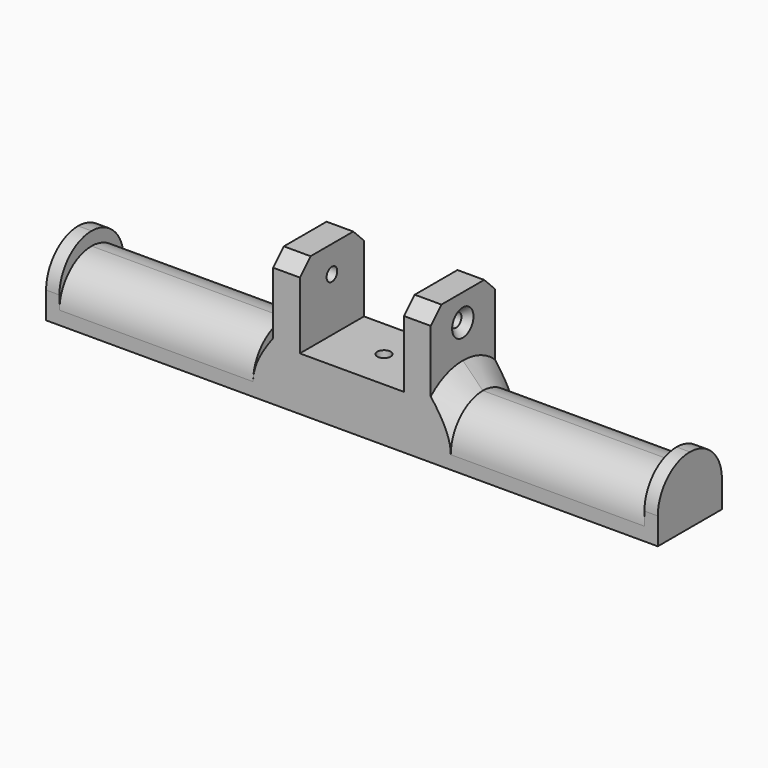
from build123d import *

# Parameters (mm, degrees)
F1_DEPTH     = 30
F2_R         = 14.99999
F4_DEPTH     = 219.001
F5_T1_DEPTH  = 2e-05
F5_T6_ANGLE  = 163.702935025
F5_T12_ANGLE = 163.702935025
F5_T18_ANGLE = 163.702935025
F5_T24_ANGLE = 163.702935025
F6_SIZE      = 5
F7_R         = 2.5
F8_DEPTH     = 139.001
F9_W         = 20
F9_H         = 20
F11_R        = 2.5
F12_DEPTH    = 20.001
F13_SIZE     = 2.5
F14_W        = 5
F14_H        = 25
F15_DEPTH    = 30
F16_R        = 14.99999
F17_R        = 5
F18_DEPTH    = 7.5
F19_SIZE     = 2.49999


# Not quite as in the source:
# - a fillet or chamfer that OpenCascade refuses, or shapes differently, is made with other operations: its cross-section is extruded or revolved along the edge and cut away or added
# - a fillet or chamfer is up to 0.001 mm smaller than in the source, because OpenCascade refuses the exact size


with BuildPart() as f1:
    # F0 (on Front) → F1 (new body)
    with BuildSketch(Plane.XZ):
        Polygon((-109.5, 0), (0, 0), (109.5, 0), (109.5, 20), (29.5, 20), (29.5, 50), (19.5, 50), (19.5, 20), (0, 20), (-19.5, 20), (-19.5, 50), (-29.5, 50), (-29.5, 20), (-109.5, 20), align=None)
    extrude(amount=F1_DEPTH)

    # F2 (radius 15 in the source; OpenCascade refuses exactly that, so slightly less here)
    f2_edges = [f1.edges().sort_by_distance(p)[0] for p in [
        (-69.5, 0, 20),
        (-69.5, -30, 20),
        (69.5, 0, 20),
        (69.5, -30, 20),
    ]]
    fillet(f2_edges, radius=F2_R)

    # F3 (on face) → F4 (cut, through all)
    with BuildSketch(Plane(origin=(-109.5, 0, 0), x_dir=(0, -1, 0), z_dir=(-1, 0, 0))):
        with BuildLine():
            Line((25, 0), (25, 5))
            ThreePointArc((25, 5), (15, 15), (5, 5))
            Line((5, 5), (5, 0))
            Line((5, 0), (25, 0))
        make_face()
    extrude(amount=-F4_DEPTH, mode=Mode.SUBTRACT)

    # F5: chamfer of 7.5 on 4 edges, made by hand

    # F5_s2 → F5_t1 (join)
    with BuildSketch(Plane.XZ.offset(14.99999)):
        Polygon((-37, 20), (-29.5, 27.5), (-29.5, 20), align=None)
        Polygon((37, 20), (29.5, 27.5), (29.5, 20), align=None)
    extrude(amount=F5_T1_DEPTH)


with BuildPart() as f5_tool4:
    # F5_s5 → F5_t6 (revolve)
    with BuildSketch(Plane(origin=(0, -12.4720838446, -3.6463990318), x_dir=(1, 0, 0), z_dir=(0, -0.9598196681, -0.2806175417))):
        Polygon((-37, -5.9916217418), (-29.5, -13.4916217418), (-29.5, -5.9916217418), align=None)
    revolve(axis=Axis((-29.5, -14.99999, 5.00001), (1, 0, 0)), revolution_arc=F5_T6_ANGLE)

    split(bisect_by=Plane.XZ, keep=Keep.TOP)

    split(bisect_by=Plane.XY, keep=Keep.TOP)


with BuildPart() as f1_1:
    add(f1.part)

    # F5_t3: union F5_tool4
    add(f5_tool4.part)


with BuildPart() as f5_tool10:
    # F5_s11 → F5_t12 (revolve)
    with BuildSketch(Plane(origin=(0, -12.4720838446, -3.6463990318), x_dir=(1, 0, 0), z_dir=(0, -0.9598196681, -0.2806175417))):
        Polygon((29.5, -13.4916217418), (37, -5.9916217418), (29.5, -5.9916217418), align=None)
    revolve(axis=Axis((29.5, -14.99999, 5.00001), (1, 0, 0)), revolution_arc=F5_T12_ANGLE)

    split(bisect_by=Plane.XZ, keep=Keep.TOP)

    split(bisect_by=Plane.XY, keep=Keep.TOP)


with BuildPart() as f1_2:
    add(f1_1.part)

    # F5_t9: union F5_tool10
    add(f5_tool10.part)


with BuildPart() as f5_tool16:
    # F5_s17 → F5_t18 (revolve)
    with BuildSketch(Plane.XZ.offset(15.00001)):
        Polygon((37, 20), (29.5, 27.5), (29.5, 20), align=None)
    revolve(axis=Axis((29.5, -15.00001, 5.00001), (1, 0, 0)), revolution_arc=F5_T18_ANGLE)

    split(bisect_by=Plane.XY, keep=Keep.TOP)

    split(bisect_by=Plane.XZ.offset(30), keep=Keep.BOTTOM)


with BuildPart() as f1_3:
    add(f1_2.part)

    # F5_t15: union F5_tool16
    add(f5_tool16.part)


with BuildPart() as f5_tool22:
    # F5_s23 → F5_t24 (revolve)
    with BuildSketch(Plane.XZ.offset(15.00001)):
        Polygon((-37, 20), (-29.5, 27.5), (-29.5, 20), align=None)
    revolve(axis=Axis((-29.5, -15.00001, 5.00001), (1, 0, 0)), revolution_arc=F5_T24_ANGLE)

    split(bisect_by=Plane.XY, keep=Keep.TOP)

    split(bisect_by=Plane.XZ.offset(30), keep=Keep.BOTTOM)


with BuildPart() as f1_4:
    add(f1_3.part)

    # F5_t21: union F5_tool22
    add(f5_tool22.part)

    # F6
    f6_edges = [f1_4.edges().sort_by_distance(p)[0] for p in [
        (-24.5, 0, 50),
        (-24.5, -30, 50),
        (24.5, 0, 50),
        (24.5, -30, 50),
    ]]
    chamfer(f6_edges, length=F6_SIZE)

    # F7 (on face) → F8 (cut, through all)
    with BuildSketch(Plane.YZ.offset(29.5)):
        with Locations((-15, 40)):
            Circle(F7_R)
    extrude(amount=-F8_DEPTH, mode=Mode.SUBTRACT)

    # F9 (on face) → F10 (join, up to the next surface of F1)
    with BuildSketch(Plane(origin=(0, 0, 0), x_dir=(1, 0, 0), z_dir=(0, 0, -1))):
        with Locations((0, 15)):
            Rectangle(F9_W, F9_H)
    extrude(until=Until.NEXT, dir=(0, 0, 1))

    # F11 (on face) → F12 (cut, through all)
    with BuildSketch(Plane.XY.offset(20)):
        with Locations((0, -15)):
            Circle(F11_R)
    extrude(amount=-F12_DEPTH, mode=Mode.SUBTRACT)

    # F13
    f13_edges = [f1_4.edges().sort_by_distance(p)[0] for p in [
        (-29.5, -17.5, 40),
        (29.5, -17.5, 40),
    ]]
    chamfer(f13_edges, length=F13_SIZE)

    # F14 (on face) → F15 (join, through all)
    with BuildSketch(Plane.XZ.offset(30)):
        with Locations((-112, 12.5)):
            Rectangle(F14_W, F14_H)
        with Locations((112, 12.5)):
            Rectangle(F14_W, F14_H)
    extrude(amount=-F15_DEPTH)

    # F16 (radius 15 in the source; OpenCascade refuses exactly that, so slightly less here)
    f16_edges = [f1_4.edges().sort_by_distance(p)[0] for p in [
        (112, 0, 25),
        (112, -30, 25),
        (-112, -30, 25),
        (-112, 0, 25),
    ]]
    fillet(f16_edges, radius=F16_R)

    # F17 (on face) → F18 (cut)
    with BuildSketch(Plane(origin=(0, 0, 0), x_dir=(1, 0, 0), z_dir=(0, 0, -1))):
        with Locations((0, 15)):
            Circle(F17_R)
    extrude(amount=-F18_DEPTH, mode=Mode.SUBTRACT)

    # F19 (size 2.5 in the source; OpenCascade refuses exactly that, so slightly less here)
    f19_edges = [f1_4.edges().sort_by_distance(p)[0] for p in [
        (-2.5, -15, 7.5),
    ]]
    chamfer(f19_edges, length=F19_SIZE)


solid = f1_4.part
